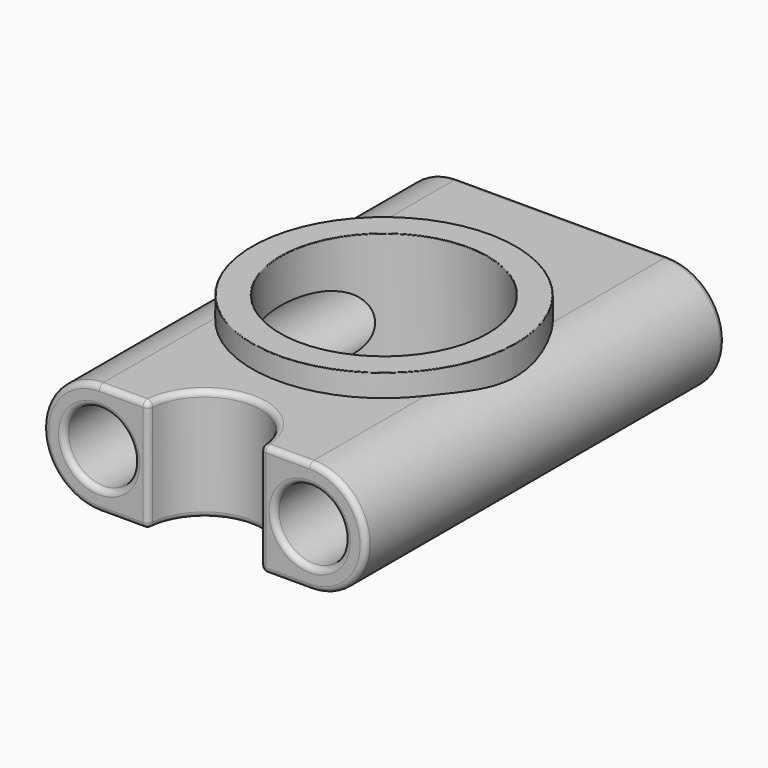
from build123d import *

# Parameters (mm, degrees)
F0_R     = 7.9375
F1_DEPTH = 50.8
F2_R     = 12.7
F3_DEPTH = 25.401
F4_R     = 23.495
F4_R_2   = 12.7
F5_DEPTH = 22.86
F6_R     = 19.05
F6_R_2   = 12.7
F7_DEPTH = 5.08
F9_DEPTH = 25.4010001
F10_R    = 1.27
F12_R    = 29.845
F12_R_2  = 23.495
F14_R    = 0.127


# Not quite as in the source:
# - a feature names something its author has since deleted; it is built from what else it names


with BuildPart() as f1:
    # F0 (on Front) → F1 (new body, symmetric)
    with BuildSketch(Plane.XZ):
        with BuildLine():
            ThreePointArc((-23.8125, 12.7), (-36.5125, 0), (-23.8125, -12.7))
            Line((-23.8125, -12.7), (0, -12.7))
            Line((0, -12.7), (0, 12.7))
            Line((0, 12.7), (-23.8125, 12.7))
        make_face()
        with Locations((-23.8125, 0)):
            Circle(F0_R, mode=Mode.SUBTRACT)
        with BuildLine():
            Line((0, 12.7), (0, -12.7))
            Line((0, -12.7), (23.8125, -12.7))
            ThreePointArc((23.8125, -12.7), (36.5125, 0), (23.8125, 12.7))
            Line((23.8125, 12.7), (0, 12.7))
        make_face()
        with Locations((23.8125, 0)):
            Circle(F0_R, mode=Mode.SUBTRACT)
    extrude(amount=F1_DEPTH, both=True)

    # F2 (on face) → F3 (cut, through all)
    with BuildSketch(Plane.XY.offset(12.7)):
        Circle(F2_R)
    extrude(amount=-F3_DEPTH, mode=Mode.SUBTRACT)

    # F4 (on face) → F5 (cut)
    with BuildSketch(Plane.XY.offset(12.7)):
        Circle(F4_R)
        Circle(F4_R_2, mode=Mode.SUBTRACT)
    extrude(amount=-F5_DEPTH, mode=Mode.SUBTRACT)

    # F6 (on face) → F7 (join)
    with BuildSketch(Plane(origin=(0, 0, -12.7), x_dir=(1, 0, 0), z_dir=(0, 0, -1))):
        Circle(F6_R)
        Circle(F6_R_2, mode=Mode.SUBTRACT)
    extrude(amount=F7_DEPTH)

    # F8 (on face) → F9 (cut, through all)
    with BuildSketch(Plane(origin=(0, 0, -12.7), x_dir=(1, 0, 0), z_dir=(0, 0, -1))):
        with BuildLine():
            Line((12.7, 50.8), (-12.7, 50.8))
            ThreePointArc((-12.7, 50.8), (0, 38.1), (12.7, 50.8))
        make_face()
    extrude(amount=-F9_DEPTH, mode=Mode.SUBTRACT)

    # F10
    f10_edges = [f1.edges().sort_by_distance(p)[0] for p in [
        (0, 50.8, 12.7),
        (-36.5125, -50.8, 0),
        (-18.25625, -50.8, 12.7),
        (-12.7, -50.8, 0),
        (-18.25625, -50.8, -12.7),
        (-31.75, -50.8, 0),
        (12.7, -50.8, 0),
        (18.25625, -50.8, 12.7),
        (36.5125, -50.8, 0),
        (18.25625, -50.8, -12.7),
        (15.875, -50.8, 0),
        (0, -38.1, -12.7),
        (0, -38.1, 12.7),
        (15.875, 50.8, 0),
        (-31.75, 50.8, 0),
    ]]
    fillet(f10_edges, radius=F10_R)

    # F12 (on offset) → F13 (join, up to the next surface of F1)
    with BuildSketch(Plane.XY.offset(17.78)):
        Circle(F12_R)
        Circle(F12_R_2, mode=Mode.SUBTRACT)
    extrude(until=Until.NEXT, dir=(0, 0, -1))

    # F14
    f14_edges = [f1.edges().sort_by_distance(p)[0] for p in [
        (-29.845, 0, 17.78),
        (-23.495, 0, 17.78),
        (-19.05, 0, -17.78),
    ]]
    fillet(f14_edges, radius=F14_R)


solid = f1.part
